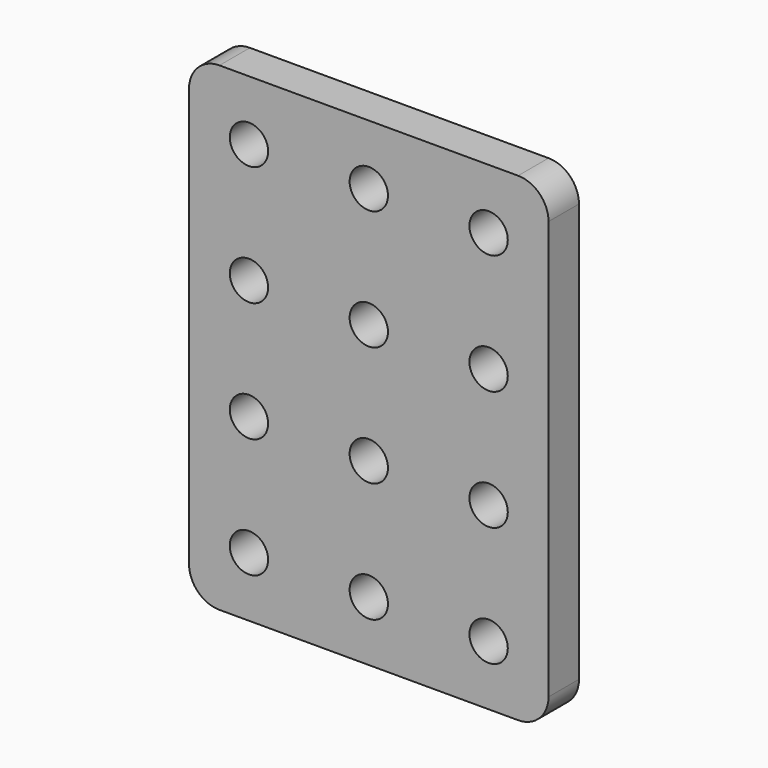
from build123d import *

# Parameters (mm, degrees)
F0_R     = 1.6
F1_DEPTH = 3.175


# Not quite as in the source:
# - a length typed as a fraction of an inch, garbled in the dataset ("3 / 203.2 mm" for 3/8 in), is restored


with BuildPart() as f1:
    # F0 (on Front) → F1 (new body)
    with BuildSketch(Plane.XZ):
        with BuildLine():
            Line((27.46, 0), (2.54, 0))
            ThreePointArc((2.54, 0), (0.7439487758, -0.7439487758), (0, -2.54))
            Line((0, -2.54), (0, -37.46))
            ThreePointArc((0, -37.46), (0.7439487758, -39.2560512242), (2.54, -40))
            Line((2.54, -40), (27.46, -40))
            ThreePointArc((27.46, -40), (29.2560512242, -39.2560512242), (30, -37.46))
            Line((30, -37.46), (30, -2.54))
            ThreePointArc((30, -2.54), (29.2560512242, -0.7439487758), (27.46, 0))
        make_face()
        with Locations((5, -35)):
            Circle(F0_R, mode=Mode.SUBTRACT)
        with Locations((5, -25)):
            Circle(F0_R, mode=Mode.SUBTRACT)
        with Locations((15, -35)):
            Circle(F0_R, mode=Mode.SUBTRACT)
        with Locations((25, -35)):
            Circle(F0_R, mode=Mode.SUBTRACT)
        with Locations((15, -25)):
            Circle(F0_R, mode=Mode.SUBTRACT)
        with Locations((25, -25)):
            Circle(F0_R, mode=Mode.SUBTRACT)
        with Locations((5, -15)):
            Circle(F0_R, mode=Mode.SUBTRACT)
        with Locations((5, -5)):
            Circle(F0_R, mode=Mode.SUBTRACT)
        with Locations((15, -15)):
            Circle(F0_R, mode=Mode.SUBTRACT)
        with Locations((25, -15)):
            Circle(F0_R, mode=Mode.SUBTRACT)
        with Locations((15, -5)):
            Circle(F0_R, mode=Mode.SUBTRACT)
        with Locations((25, -5)):
            Circle(F0_R, mode=Mode.SUBTRACT)
    extrude(amount=F1_DEPTH)


solid = f1.part
